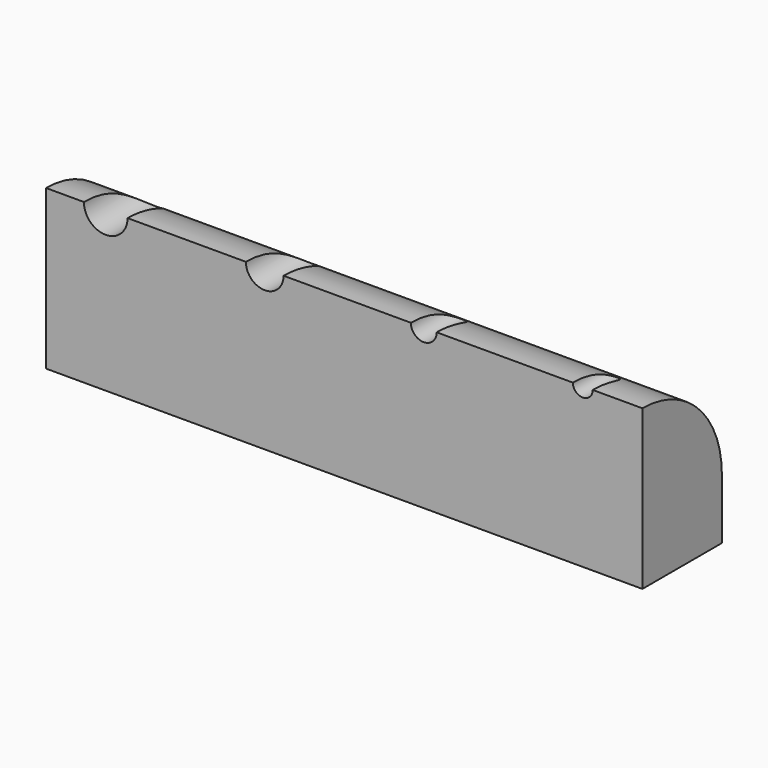
from build123d import *

# Parameters (mm, degrees)
F0_W     = 38.1
F0_H     = 6.35
F1_DEPTH = 10.16
F2_R     = 6.34999
F4_DEPTH = 25.4


# Not quite as in the source:
# - a fillet or chamfer is up to 0.001 mm smaller than in the source, because OpenCascade refuses the exact size


with BuildPart() as f1:
    # F0 (on Top) → F1 (new body)
    with BuildSketch(Plane.XY):
        with Locations((0, 3.175)):
            Rectangle(F0_W, F0_H)
    extrude(amount=F1_DEPTH)

    # F2 (radius 6.35 in the source; OpenCascade refuses exactly that, so slightly less here)
    f2_edges = [f1.edges().sort_by_distance(p)[0] for p in [
        (0, 6.35, 10.16),
    ]]
    fillet(f2_edges, radius=F2_R)

    # F3 (on face) → F4 (cut)
    with BuildSketch(Plane.XZ):
        with BuildLine():
            ThreePointArc((-16.637, 10.16), (-15.24, 8.763), (-13.843, 10.16))
            Line((-13.843, 10.16), (-16.637, 10.16))
        make_face()
        with BuildLine():
            Line((-3.8735, 10.16), (-6.2865, 10.16))
            ThreePointArc((-6.2865, 10.16), (-5.08, 8.9535), (-3.8735, 10.16))
        make_face()
        with BuildLine():
            Line((5.9055, 10.16), (4.2545, 10.16))
            ThreePointArc((4.2545, 10.16), (5.08, 9.3345), (5.9055, 10.16))
        make_face()
        with BuildLine():
            Line((15.875, 10.16), (14.605, 10.16))
            ThreePointArc((14.605, 10.16), (15.24, 9.525), (15.875, 10.16))
        make_face()
    extrude(amount=-F4_DEPTH, mode=Mode.SUBTRACT)


solid = f1.part
